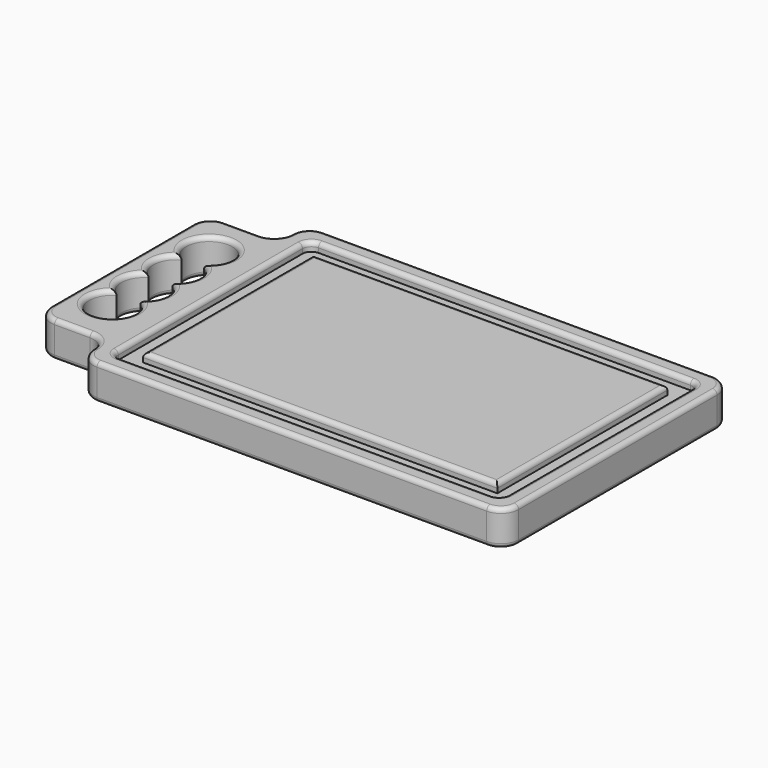
from build123d import *

# Parameters (mm, degrees)
F0_W     = 50.8
F0_H     = 152.4
F1_DEPTH = 25.4
F4_DEPTH = 25.4
F5_W     = 254
F5_H     = 152.4
F6_DEPTH = 6.35
F7_R     = 6.35
F8_R     = 12.69999
F9_R     = 3.175


# Not quite as in the source:
# - a fillet or chamfer is up to 0.001 mm smaller than in the source, because OpenCascade refuses the exact size


with BuildPart() as f1:
    # F0 (on Top) → F1 (new body)
    with BuildSketch(Plane.XY):
        Polygon((0, 25.4), (0, 0), (304.8, 0), (304.8, 203.2), (0, 203.2), (0, 177.8), align=None)
        with Locations((-25.4, 101.6)):
            Rectangle(F0_W, F0_H)
    extrude(amount=F1_DEPTH)

    # F2 (on face) + F3 (on face) → F4 (cut)
    with BuildSketch(Plane.XY.offset(25.4)):
        with BuildLine():
            ThreePointArc((-15.2907530688, 102.525351261), (-7.2065932651, 116.6708042855), (-15.2003335319, 130.8675503052))
            ThreePointArc((-15.2003335319, 130.8675503052), (-22.8489691097, 161.8355395984), (-31.6825862945, 131.1845168667))
            ThreePointArc((-31.6825862945, 131.1845168667), (-40.2160226994, 117.3118256345), (-32.6923659242, 102.8665604024))
            ThreePointArc((-32.6923659242, 102.8665604024), (-40.7734367687, 88.9921051486), (-33.2424743946, 74.8115261652))
            ThreePointArc((-33.2424743946, 74.8115261652), (-25.1403717333, 44.1065805763), (-15.840843765, 74.470317677))
            ThreePointArc((-15.840843765, 74.470317677), (-7.7597825179, 88.3447775601), (-15.2907530688, 102.525351261))
        make_face()
    with BuildSketch(Plane.XY):
        with BuildLine():
            ThreePointArc((-15.2003335319, 130.8675503052), (-22.8489691097, 161.8355395984), (-31.6825862945, 131.1845168667))
            ThreePointArc((-31.6825862945, 131.1845168667), (-40.2160226994, 117.3118256345), (-32.6923659242, 102.8665604024))
            ThreePointArc((-32.6923659242, 102.8665604024), (-40.7734367687, 88.9921051486), (-33.2424743946, 74.8115261652))
            ThreePointArc((-33.2424743946, 74.8115261652), (-25.1403717333, 44.1065805763), (-15.840843765, 74.470317677))
            ThreePointArc((-15.840843765, 74.470317677), (-7.7597825179, 88.3447775601), (-15.2907530688, 102.525351261))
            ThreePointArc((-15.2907530688, 102.525351261), (-7.2065932651, 116.6708042855), (-15.2003335319, 130.8675503052))
        make_face()
    extrude(amount=-F4_DEPTH, mode=Mode.SUBTRACT)

    # F5 (on face) → F6 (cut)
    with BuildSketch(Plane.XY.offset(25.4)):
        Polygon((12.7, 25.4), (12.7, 12.7), (292.1, 12.7), (292.1, 190.5), (12.7, 190.5), (12.7, 177.8), align=None)
        with Locations((152.4, 101.6)):
            Rectangle(F5_W, F5_H, mode=Mode.SUBTRACT)
    extrude(amount=-F6_DEPTH, mode=Mode.SUBTRACT)

    # F7
    f7_edges = [f1.edges().sort_by_distance(p)[0] for p in [
        (12.7, 190.5, 22.225),
        (292.1, 190.5, 22.225),
        (292.1, 12.7, 22.225),
        (12.7, 12.7, 22.225),
    ]]
    fillet(f7_edges, radius=F7_R)

    # F8 (radius 12.7 in the source; OpenCascade refuses exactly that, so slightly less here)
    f8_edges = [f1.edges().sort_by_distance(p)[0] for p in [
        (304.8, 0, 12.7),
        (304.8, 203.2, 12.7),
        (0, 0, 12.7),
        (-50.8, 25.4, 12.7),
        (0, 25.4, 12.7),
        (-50.8, 177.8, 12.7),
        (0, 177.8, 12.7),
        (0, 203.2, 12.7),
    ]]
    fillet(f8_edges, radius=F8_R)

    # F9
    f9_edges = [f1.edges().sort_by_distance(p)[0] for p in [
        (152.4, 25.4, 25.4),
        (25.4, 101.6, 25.4),
        (152.4, 177.8, 25.4),
        (279.4, 101.6, 25.4),
        (0, 190.5, 25.4),
        (3.719741, 199.480259, 25.4),
        (-3.719741, 181.519741, 25.4),
        (152.4, 203.2, 25.4),
        (-25.4, 177.8, 25.4),
        (301.080259, 199.480259, 25.4),
        (-47.080259, 174.080259, 25.4),
        (304.8, 101.6, 25.4),
        (-50.8, 101.6, 25.4),
        (301.080259, 3.719741, 25.4),
        (-47.080259, 29.119741, 25.4),
        (152.4, 0, 25.4),
        (-25.4, 25.4, 25.4),
        (3.719741, 3.719741, 25.4),
        (-3.719741, 21.680259, 25.4),
        (0, 12.7, 25.4),
        (152.4, 12.7, 25.4),
        (14.559872, 14.559872, 25.4),
        (290.240128, 14.559872, 25.4),
        (12.7, 101.6, 25.4),
        (292.1, 101.6, 25.4),
        (14.559872, 188.640128, 25.4),
        (290.240128, 188.640128, 25.4),
        (152.4, 190.5, 25.4),
        (-7.206593, 116.670804, 25.4),
        (-7.759783, 88.344778, 25.4),
        (-22.848969, 161.83554, 25.4),
        (-25.140372, 44.106581, 25.4),
        (-40.216023, 117.311826, 25.4),
        (-40.773437, 88.992105, 25.4),
        (0, 190.5, 0),
        (3.719741, 199.480259, 0),
        (-3.719741, 181.519741, 0),
        (152.4, 203.2, 0),
        (-25.4, 177.8, 0),
        (301.080259, 199.480259, 0),
        (-47.080259, 174.080259, 0),
        (304.8, 101.6, 0),
        (-50.8, 101.6, 0),
        (301.080259, 3.719741, 0),
        (-47.080259, 29.119741, 0),
        (152.4, 0, 0),
        (-25.4, 25.4, 0),
        (3.719741, 3.719741, 0),
        (-3.719741, 21.680259, 0),
        (0, 12.7, 0),
        (-7.206593, 116.670804, 0),
        (-22.848969, 161.83554, 0),
        (-40.216023, 117.311826, 0),
        (-40.773437, 88.992105, 0),
        (-25.140372, 44.106581, 0),
        (-7.759783, 88.344778, 0),
    ]]
    fillet(f9_edges, radius=F9_R)


solid = f1.part
